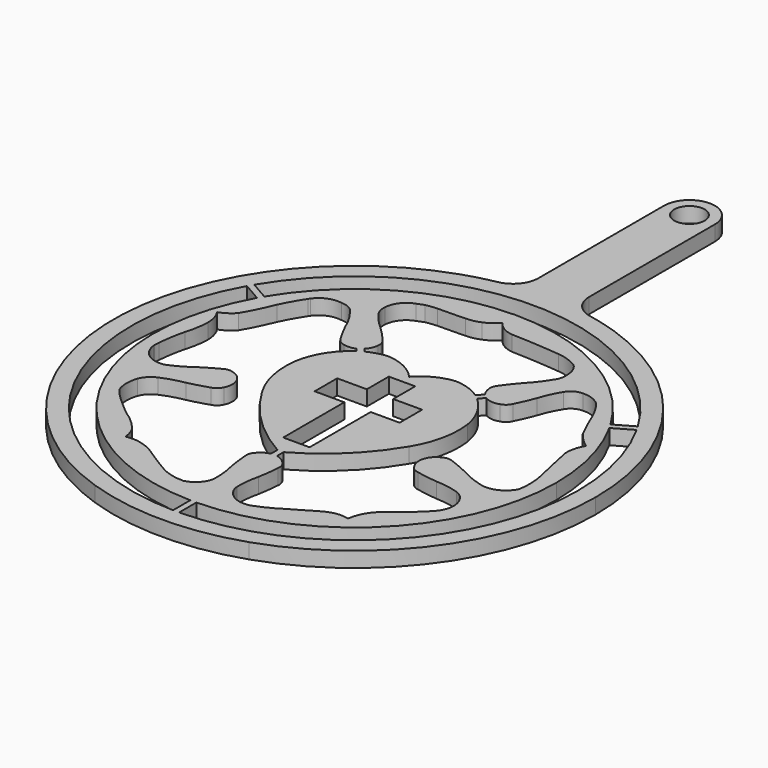
from build123d import *

# Parameters (mm, degrees)
F1_DEPTH = 3
F2_R     = 4.99999
F3_R     = 3
F4_DEPTH = 3.001


# Not quite as in the source:
# - a fillet or chamfer is up to 0.001 mm smaller than in the source, because OpenCascade refuses the exact size
# - a feature names something its author has since deleted; it is built from what else it names


with BuildPart() as f1:
    # F0 (on Top) → F1 (new body)
    with BuildSketch(Plane.XY):
        with BuildLine():
            Line((15.2069063257, 45), (-15.2069063257, 45))
            ThreePointArc((-15.2069063257, 45), (-33.5875721064, 33.5875721064), (-45, 15.2069063257))
            Line((-45, 15.2069063257), (-45, -15.2069063257))
            ThreePointArc((-45, -15.2069063257), (-33.5875721064, -33.5875721064), (-15.2069063257, -45))
            Line((-15.2069063257, -45), (15.2069063257, -45))
            ThreePointArc((15.2069063257, -45), (33.5875721064, -33.5875721064), (45, -15.2069063257))
            Line((45, -15.2069063257), (45, 15.2069063257))
            ThreePointArc((45, 15.2069063257), (33.5875721064, 33.5875721064), (15.2069063257, 45))
        make_face()
        with BuildLine():
            ThreePointArc((38.4015747706, 21.4783392081), (42.5773959391, 11.0979887839), (44, 0))
            ThreePointArc((44, 0), (31.3241121183, -30.8998381873), (0.6, -43.9959089007))
            ThreePointArc((0.6, -43.9959089007), (0, -44), (-0.6, -43.9959089007))
            ThreePointArc((-0.6, -43.9959089007), (-38.1051177665, -22), (-38.4015747706, 21.4783392081))
            ThreePointArc((-38.4015747706, 21.4783392081), (-38.1051177665, 22), (-37.8015747706, 22.5175696926))
            ThreePointArc((-37.8015747706, 22.5175696926), (0, 44), (37.8015747706, 22.5175696926))
            ThreePointArc((37.8015747706, 22.5175696926), (38.1051177665, 22), (38.4015747706, 21.4783392081))
        make_face(mode=Mode.SUBTRACT)
        with BuildLine():
            ThreePointArc((39.75, 0), (38.4721059413, 9.9979780177), (34.7205879526, 19.3531204778))
            ThreePointArc((34.7205879526, 19.3531204778), (34.4245098004, 19.875), (34.1205879526, 20.3923509623))
            ThreePointArc((34.1205879526, 20.3923509623), (0, 39.75), (-34.1205879526, 20.3923509623))
            ThreePointArc((-34.1205879526, 20.3923509623), (-34.4245098004, 19.875), (-34.7205879526, 19.3531204778))
            ThreePointArc((-34.7205879526, 19.3531204778), (-34.4245098004, -19.875), (-0.6, -39.7454714402))
            ThreePointArc((-0.6, -39.7454714402), (0, -39.75), (0.6, -39.7454714402))
            ThreePointArc((0.6, -39.7454714402), (28.3188320734, -27.8945559205), (39.75, 0))
        make_face()
        with BuildLine():
            ThreePointArc((13.1544303149, 18.6974834651), (12.9994836516, 17.710085626), (13.2698951604, 16.7478795269))
            ThreePointArc((13.2698951604, 16.7478795269), (13.6237788684, 16.2513300709), (14.0937424239, 15.8628338707))
            ThreePointArc((14.0937424239, 15.8628338707), (15.8973722034, 15.5715459018), (17.3623822629, 16.6631843895))
            ThreePointArc((17.3623822629, 16.6631843895), (18.3033011466, 18.6424294995), (19.0587975085, 20.6996034831))
            ThreePointArc((19.0587975085, 20.6996034831), (19.6962425586, 22.4376385334), (20.4611290246, 24.1234768182))
            ThreePointArc((20.4611290246, 24.1234768182), (21.7193319348, 25.6187652762), (23.5025491565, 26.4182016253))
            ThreePointArc((23.5025491565, 26.4182016253), (25.4580904224, 26.3810636918), (27.1545499563, 25.4076439887))
            ThreePointArc((27.1545499563, 25.4076439887), (27.52673708, 25.0168961336), (27.8844064433, 24.6128172206))
            ThreePointArc((27.8844064433, 24.6128172206), (29.2916671808, 22.6613798031), (30.363548547, 20.5074157566))
            ThreePointArc((30.363548547, 20.5074157566), (31.5171358074, 17.8349379562), (32.7894538641, 15.2169028297))
            ThreePointArc((32.7894538641, 15.2169028297), (34.1230277014, 13.7207168946), (35.6659889221, 12.4415522441))
            ThreePointArc((35.6659889221, 12.4415522441), (34.8647886426, 10.5924571906), (34.6556343138, 8.5881296545))
            ThreePointArc((34.6556343138, 8.5881296545), (35.5419764472, 4.3940722193), (36.4768467844, 0.2105644089))
            ThreePointArc((36.4768467844, 0.2105644089), (36.8063640413, -2.5236804449), (36.5942801272, -5.269531307))
            ThreePointArc((36.5942801272, -5.269531307), (36.5776420507, -5.3615212162), (36.5603901446, -5.4533979855))
            ThreePointArc((36.5603901446, -5.4533979855), (35.5463694507, -7.1539827552), (34.0106971562, -8.4037575871))
            ThreePointArc((34.0106971562, -8.4037575871), (32.5922946208, -8.674299863), (31.1614554375, -8.4799854085))
            ThreePointArc((31.1614554375, -8.4799854085), (27.7166740101, -7.1552393182), (24.3694968522, -5.6002871133))
            ThreePointArc((24.3694968522, -5.6002871133), (22.9198378539, -5.167220158), (21.4094873518, -5.2560996264))
            ThreePointArc((21.4094873518, -5.2560996264), (20.4460224679, -5.7761838724), (19.8262277991, -6.6787395626))
            ThreePointArc((19.8262277991, -6.6787395626), (19.6988373955, -7.9117885325), (20.3195624053, -8.9847929776))
            ThreePointArc((20.3195624053, -8.9847929776), (21.6411737408, -9.7871390742), (23.1533683836, -10.1091377437))
            ThreePointArc((23.1533683836, -10.1091377437), (25.0267759883, -10.2520123025), (26.8935356289, -10.4647977278))
            ThreePointArc((26.8935356289, -10.4647977278), (28.7622135844, -10.6241884707), (30.5648632348, -11.1416988075))
            ThreePointArc((30.5648632348, -11.1416988075), (31.9095412868, -12.2463559177), (32.7662372269, -13.7611161168))
            ThreePointArc((32.7662372269, -13.7611161168), (32.8659343413, -15.4387331126), (32.3565080762, -17.040239647))
            ThreePointArc((32.3565080762, -17.040239647), (31.9517024959, -17.7441363632), (31.4918024275, -18.4133374331))
            ThreePointArc((31.4918024275, -18.4133374331), (30.8813307917, -19.1535972301), (30.2035380155, -19.8327563703))
            ThreePointArc((30.2035380155, -19.8327563703), (28.6944924477, -21.2622272709), (27.0892698318, -22.5827824324))
            ThreePointArc((27.0892698318, -22.5827824324), (25.8109799054, -23.5447087894), (24.6124230325, -24.6043261141))
            ThreePointArc((24.6124230325, -24.6043261141), (23.0161745176, -26.6759411416), (22.1902150661, -29.1573498398))
            ThreePointArc((22.1902150661, -29.1573498398), (22.1823714034, -29.2604491115), (22.1902150661, -29.3635483831))
            ThreePointArc((22.1902150661, -29.3635483831), (20.6543600705, -29.1355721936), (19.1159117967, -29.3453354388))
            ThreePointArc((19.1159117967, -29.3453354388), (18.0140299323, -29.7476012069), (16.9789958745, -30.2995666862))
            ThreePointArc((16.9789958745, -30.2995666862), (14.8518935693, -31.5584511018), (12.7147845924, -32.8002721071))
            ThreePointArc((12.7147845924, -32.8002721071), (10.3373434694, -34.1802416761), (7.8145563602, -35.2720692754))
            ThreePointArc((7.8145563602, -35.2720692754), (4.7183466369, -35.6236947606), (1.902480959, -34.2891328037))
            ThreePointArc((1.902480959, -34.2891328037), (1.1117117622, -32.5153233248), (1.0741840815, -30.5735953152))
            ThreePointArc((1.0741840815, -30.5735953152), (1.4077427625, -27.3798938968), (1.8937365385, -24.2058113217))
            ThreePointArc((1.8937365385, -24.2058113217), (1.9589663636, -22.7965979751), (1.7485594144, -21.4016549289))
            ThreePointArc((1.7485594144, -21.4016549289), (1.3000904024, -20.7086359573), (0.6, -20.2712880658))
            ThreePointArc((0.6, -20.2712880658), (0.3043633322, -20.1930320032), (0, -20.1632324606))
            ThreePointArc((0, -20.1632324606), (-0.3001138701, -20.1435719399), (-0.6, -20.1664450732))
            ThreePointArc((-0.6, -20.1664450732), (-1.5074907875, -20.5274222481), (-2.1579356398, -21.2559588253))
            ThreePointArc((-2.1579356398, -21.2559588253), (-2.5611237062, -22.7415693157), (-2.4770193268, -24.278620258))
            ThreePointArc((-2.4770193268, -24.278620258), (-1.9152687902, -27.3259041519), (-1.5005924506, -30.3966607898))
            ThreePointArc((-1.5005924506, -30.3966607898), (-1.7771048177, -32.3321939483), (-2.8084376827, -33.9932478964))
            ThreePointArc((-2.8084376827, -33.9932478964), (-3.8656823021, -34.9221705279), (-5.2103865892, -35.3374220431))
            ThreePointArc((-5.2103865892, -35.3374220431), (-5.344161676, -35.3425806413), (-5.4779952594, -35.3458907678))
            ThreePointArc((-5.4779952594, -35.3458907678), (-7.7809432718, -35.1103947403), (-9.962332435, -34.3354307115))
            ThreePointArc((-9.962332435, -34.3354307115), (-12.6447845502, -32.7277147455), (-15.2711598203, -31.0299359262))
            ThreePointArc((-15.2711598203, -31.0299359262), (-16.8965931087, -30.0854125724), (-18.6754819006, -29.4773727655))
            ThreePointArc((-18.6754819006, -29.4773727655), (-20.163660707, -29.2771457572), (-21.6584373266, -29.4200088829))
            ThreePointArc((-21.6584373266, -29.4200088829), (-21.9469277164, -27.9249853374), (-22.6042401046, -26.551572606))
            ThreePointArc((-22.6042401046, -26.551572606), (-24.4508663247, -24.6630203424), (-26.5681687742, -23.0838786811))
            ThreePointArc((-26.5681687742, -23.0838786811), (-28.2946605833, -21.6202528417), (-29.9907564706, -20.1215089324))
            ThreePointArc((-29.9907564706, -20.1215089324), (-31.1955319716, -18.9227074216), (-32.2594381869, -17.5972970567))
            ThreePointArc((-32.2594381869, -17.5972970567), (-32.7127552743, -16.9261962228), (-33.1298090107, -16.2319780353))
            ThreePointArc((-33.1298090107, -16.2319780353), (-33.5060127096, -14.1649201538), (-33.1298090107, -12.0978622723))
            ThreePointArc((-33.1298090107, -12.0978622723), (-31.9416458989, -10.6809065614), (-30.2762478179, -9.8771999615))
            ThreePointArc((-30.2762478179, -9.8771999615), (-27.3934880183, -9.0605324957), (-24.4824323392, -8.3513042915))
            ThreePointArc((-24.4824323392, -8.3513042915), (-22.8843269804, -7.9189260706), (-21.4011013097, -7.1834444094))
            ThreePointArc((-21.4011013097, -7.1834444094), (-20.6895055917, -6.0012895415), (-20.7867655492, -4.6249178263))
            ThreePointArc((-20.7867655492, -4.6249178263), (-21.7066659737, -3.4710484078), (-23.1462172753, -3.1465126227))
            ThreePointArc((-23.1462172753, -3.1465126227), (-25.0854890454, -3.7516390034), (-26.8341671265, -4.7856012385))
            ThreePointArc((-26.8341671265, -4.7856012385), (-28.4361773324, -5.8823391866), (-30.0850268043, -6.9073105256))
            ThreePointArc((-30.0850268043, -6.9073105256), (-31.4989957357, -7.5753525343), (-33.0535970218, -7.7450673121))
            ThreePointArc((-33.0535970218, -7.7450673121), (-34.8285220711, -7.3095151895), (-36.249821592, -6.1606147352))
            ThreePointArc((-36.249821592, -6.1606147352), (-36.9862452296, -4.5062677921), (-37.2370698922, -2.7128714134))
            ThreePointArc((-37.2370698922, -2.7128714134), (-37.2194603589, -2.241264003), (-37.167636264, -1.7721820182))
            ThreePointArc((-37.167636264, -1.7721820182), (-36.8335814434, 0.9244367586), (-36.2805403358, 3.584792183))
            ThreePointArc((-36.2805403358, 3.584792183), (-35.7282804227, 5.8900650394), (-35.5035714394, 8.2498912674))
            ThreePointArc((-35.5035714394, 8.2498912674), (-35.7673793213, 10.0960235572), (-36.5443281419, 11.7913552535))
            ThreePointArc((-36.5443281419, 11.7913552535), (-35.0440824364, 12.526502069), (-33.7808481938, 13.6198534605))
            ThreePointArc((-33.7808481938, 13.6198534605), (-32.2465790302, 16.4891609765), (-30.9187691248, 19.4596539226))
            ThreePointArc((-30.9187691248, 19.4596539226), (-29.7224672012, 21.7811291171), (-28.3643565353, 24.0118063215))
            ThreePointArc((-28.3643565353, 24.0118063215), (-28.2608924895, 24.1742639387), (-28.1508342247, 24.3323286865))
            ThreePointArc((-28.1508342247, 24.3323286865), (-27.9161509949, 24.6764245366), (-27.6775840259, 25.017839202))
            ThreePointArc((-27.6775840259, 25.017839202), (-26.0121072138, 26.4235192892), (-23.9492948688, 27.1267651555))
            ThreePointArc((-23.9492948688, 27.1267651555), (-22.683343624, 27.1559317042), (-21.4851997382, 26.7461336193))
            ThreePointArc((-21.4851997382, 26.7461336193), (-20.2944890997, 25.6536896702), (-19.3477306104, 24.3441577044))
            ThreePointArc((-19.3477306104, 24.3441577044), (-18.1261905857, 22.1694079096), (-16.9467623866, 19.9715348867))
            ThreePointArc((-16.9467623866, 19.9715348867), (-16.124822625, 18.3782931612), (-14.9433059207, 17.0299525347))
            ThreePointArc((-14.9433059207, 17.0299525347), (-13.9414482308, 16.5529147578), (-12.8357349956, 16.6460926139))
            ThreePointArc((-12.8357349956, 16.6460926139), (-12.432827299, 16.8427191161), (-12.0801559116, 17.1195213667))
            ThreePointArc((-12.0801559116, 17.1195213667), (-11.9641864634, 17.2253159453), (-11.855745386, 17.338814573))
            ThreePointArc((-11.855745386, 17.338814573), (-11.3489235944, 18.28613132), (-11.3304612786, 19.3603456797))
            ThreePointArc((-11.3304612786, 19.3603456797), (-11.6131657763, 20.0806167396), (-12.0245722681, 20.7359463753))
            ThreePointArc((-12.0245722681, 20.7359463753), (-13.0298005438, 21.9109290811), (-14.1447644308, 22.9823411287))
            ThreePointArc((-14.1447644308, 22.9823411287), (-15.2704276162, 23.960127427), (-16.3859091699, 24.9495133758))
            ThreePointArc((-16.3859091699, 24.9495133758), (-17.420474299, 26.17199909), (-18.1667581201, 27.588987723))
            ThreePointArc((-18.1667581201, 27.588987723), (-18.4111606757, 29.1457914028), (-18.0553290993, 30.6809637696))
            ThreePointArc((-18.0553290993, 30.6809637696), (-17.0147657832, 32.084699542), (-15.5111001804, 32.9747758806))
            ThreePointArc((-15.5111001804, 32.9747758806), (-14.3049296056, 33.3550786383), (-13.0737277589, 33.6442492729))
            ThreePointArc((-13.0737277589, 33.6442492729), (-11.9572647742, 33.8243078309), (-10.8312694356, 33.9294038713))
            ThreePointArc((-10.8312694356, 33.9294038713), (-8.1108956333, 33.9565345059), (-5.3912550211, 34.0252704918))
            ThreePointArc((-5.3912550211, 34.0252704918), (-3.9483394584, 34.1858040453), (-2.5609757286, 34.6135869622))
            ThreePointArc((-2.5609757286, 34.6135869622), (-1.1721033451, 35.3723533238), (0, 36.4357754588))
            ThreePointArc((0, 36.4357754588), (1.5528861369, 34.9900948734), (3.5677228589, 34.3253538013))
            ThreePointArc((3.5677228589, 34.3253538013), (8.4012669361, 34.1107132353), (13.2236303762, 33.7182469666))
            ThreePointArc((13.2236303762, 33.7182469666), (15.3400282605, 33.2604879218), (17.2954601791, 32.3304506325))
            ThreePointArc((17.2954601791, 32.3304506325), (17.6949809728, 32.0658775644), (18.0804952979, 31.7812822759))
            ThreePointArc((18.0804952979, 31.7812822759), (19.0718846436, 30.3757755061), (19.5259880275, 28.7168323994))
            ThreePointArc((19.5259880275, 28.7168323994), (18.9871091632, 26.7721210867), (17.8583189845, 25.0993613154))
            Line((17.8583189845, 25.0993613154), (15.5178485438, 22.0934618264))
            ThreePointArc((15.5178485438, 22.0934618264), (14.1512044305, 20.5241774551), (13.1544303149, 18.6974834651))
        make_face(mode=Mode.SUBTRACT)
        with BuildLine():
            Line((-5, 87.5), (-5, 47.2361090692))
            ThreePointArc((-5, 47.2361090692), (0, 47.5), (5, 47.2361090692))
            Line((5, 47.2361090692), (5, 87.5))
            Line((5, 87.5), (-5, 87.5))
        make_face()
        with BuildLine():
            Line((-2.4924513418, 6.1171003617), (-2.4924513418, 11.5402890369))
            Line((-2.4924513418, 11.5402890369), (0, 11.5402890369))
            Line((0, 11.5402890369), (0, 13.4395202622))
            ThreePointArc((0, 13.4395202622), (-2.9522200359, 15.7305615155), (-6.5359184518, 16.7896077037))
            ThreePointArc((-6.5359184518, 16.7896077037), (-8.6542895394, 16.4571090738), (-10.6554259019, 15.6867165363))
            ThreePointArc((-10.6554259019, 15.6867165363), (-11.1837139042, 15.3959685754), (-11.6937909943, 15.0743415363))
            ThreePointArc((-11.6937909943, 15.0743415363), (-11.8463732448, 14.9696339693), (-11.9970198721, 14.8621601984))
            ThreePointArc((-11.9970198721, 14.8621601984), (-15.269507602, 11.1829402277), (-16.9533155859, 6.5557784401))
            ThreePointArc((-16.9533155859, 6.5557784401), (-16.6901469812, 0.6933904938), (-14.4818136469, -4.7435308807))
            ThreePointArc((-14.4818136469, -4.7435308807), (-8.4346309374, -12.4175447977), (-0.6, -18.2551356018))
            ThreePointArc((-0.6, -18.2551356018), (-0.3007512971, -18.4202689289), (0, -18.582649529))
            Line((0, -18.582649529), (0, -14.4816143438))
            Line((0, -14.4816143438), (-2.4924513418, -14.4816143438))
            Line((-2.4924513418, -14.4816143438), (-2.4924513418, 0.5696658045))
            Line((-2.4924513418, 0.5696658045), (-8.3385352045, 0.5696658045))
            Line((-8.3385352045, 0.5696658045), (-8.3385352045, 6.1171003617))
            Line((-8.3385352045, 6.1171003617), (-2.4924513418, 6.1171003617))
        make_face()
        with BuildLine():
            Line((0, 13.4395202622), (0, 11.5402890369))
            Line((0, 11.5402890369), (2.7075468097, 11.5402890369))
            Line((2.7075468097, 11.5402890369), (2.7075468097, 6.1171003617))
            Line((2.7075468097, 6.1171003617), (8.4134116769, 6.1171003617))
            Line((8.4134116769, 6.1171003617), (8.4134116769, 0.5696658045))
            Line((8.4134116769, 0.5696658045), (2.7075468097, 0.5696658045))
            Line((2.7075468097, 0.5696658045), (2.7075468097, -14.4816143438))
            Line((2.7075468097, -14.4816143438), (0, -14.4816143438))
            Line((0, -14.4816143438), (0, -18.582649529))
            ThreePointArc((0, -18.582649529), (0.3007512971, -18.4202689289), (0.6, -18.2551356018))
            ThreePointArc((0.6, -18.2551356018), (8.4346309374, -12.4175447977), (14.4818136469, -4.7435308807))
            ThreePointArc((14.4818136469, -4.7435308807), (16.6901469812, 0.6933904938), (16.9533155859, 6.5557784401))
            ThreePointArc((16.9533155859, 6.5557784401), (15.5086264172, 10.7649279062), (12.7387291979, 14.2479919906))
            ThreePointArc((12.7387291979, 14.2479919906), (12.3735173621, 14.5618907382), (11.9970198721, 14.8621601984))
            ThreePointArc((11.9970198721, 14.8621601984), (11.9004435295, 14.9315356124), (11.8030605273, 14.9997740831))
            ThreePointArc((11.8030605273, 14.9997740831), (9.2945898699, 16.2628376694), (6.5359184518, 16.7896077037))
            ThreePointArc((6.5359184518, 16.7896077037), (2.9522200359, 15.7305615155), (0, 13.4395202622))
        make_face()
        with BuildLine():
            Line((-45, -15.2069063257), (-45, 15.2069063257))
            ThreePointArc((-45, 15.2069063257), (-47.5, 0), (-45, -15.2069063257))
        make_face()
        with BuildLine():
            ThreePointArc((47.5, 0), (46.8708331481, 7.7055175037), (45, 15.2069063257))
            Line((45, 15.2069063257), (45, -15.2069063257))
            ThreePointArc((45, -15.2069063257), (46.8708331481, -7.7055175037), (47.5, 0))
        make_face()
        with BuildLine():
            ThreePointArc((-5, 47.2361090692), (-10.1651272376, 46.399570992), (-15.2069063257, 45))
            Line((-15.2069063257, 45), (15.2069063257, 45))
            ThreePointArc((15.2069063257, 45), (10.1651272376, 46.399570992), (5, 47.2361090692))
            ThreePointArc((5, 47.2361090692), (0, 47.5), (-5, 47.2361090692))
        make_face()
        with BuildLine():
            Line((15.2069063257, -45), (-15.2069063257, -45))
            ThreePointArc((-15.2069063257, -45), (0, -47.5), (15.2069063257, -45))
        make_face()
        with BuildLine():
            Line((-37.2028201905, -3.0520430721), (-37.2370698922, -2.7128714134))
            ThreePointArc((-37.2370698922, -2.7128714134), (-36.9862452296, -4.5062677921), (-36.249821592, -6.1606147352))
            ThreePointArc((-36.249821592, -6.1606147352), (-34.8285220711, -7.3095151895), (-33.0535970218, -7.7450673121))
            ThreePointArc((-33.0535970218, -7.7450673121), (-31.4989957357, -7.5753525343), (-30.0850268043, -6.9073105256))
            ThreePointArc((-30.0850268043, -6.9073105256), (-28.4361773324, -5.8823391866), (-26.8341671265, -4.7856012385))
            ThreePointArc((-26.8341671265, -4.7856012385), (-25.0854890454, -3.7516390034), (-23.1462172753, -3.1465126227))
            ThreePointArc((-23.1462172753, -3.1465126227), (-21.7066659737, -3.4710484078), (-20.7867655492, -4.6249178263))
            ThreePointArc((-20.7867655492, -4.6249178263), (-20.6895055917, -6.0012895415), (-21.4011013097, -7.1834444094))
            ThreePointArc((-21.4011013097, -7.1834444094), (-22.8843269804, -7.9189260706), (-24.4824323392, -8.3513042915))
            ThreePointArc((-24.4824323392, -8.3513042915), (-27.3934880183, -9.0605324957), (-30.2762478179, -9.8771999615))
            ThreePointArc((-30.2762478179, -9.8771999615), (-31.9416458989, -10.6809065614), (-33.1298090107, -12.0978622723))
            ThreePointArc((-33.1298090107, -12.0978622723), (-33.5060127096, -14.1649201538), (-33.1298090107, -16.2319780353))
            ThreePointArc((-33.1298090107, -16.2319780353), (-32.7127552743, -16.9261962228), (-32.2594381869, -17.5972970567))
            ThreePointArc((-32.2594381869, -17.5972970567), (-32.6321128417, -15.3758618232), (-32.2594381869, -13.1544265896))
            ThreePointArc((-32.2594381869, -13.1544265896), (-31.3761557144, -11.7768380517), (-30.011004529, -10.8744521324))
            ThreePointArc((-30.011004529, -10.8744521324), (-27.829629741, -10.0706684601), (-25.5653052745, -9.5440767125))
            ThreePointArc((-25.5653052745, -9.5440767125), (-23.545938443, -9.0389737836), (-21.558195876, -8.421032964))
            ThreePointArc((-21.558195876, -8.421032964), (-20.6612270025, -7.9549542831), (-20.0762329553, -7.1305972844))
            ThreePointArc((-20.0762329553, -7.1305972844), (-19.9343099504, -4.2114197585), (-22.1327785323, -2.2856795213))
            ThreePointArc((-22.1327785323, -2.2856795213), (-23.1321423428, -2.133842533), (-24.0904982241, -2.4553024864))
            ThreePointArc((-24.0904982241, -2.4553024864), (-25.9158096623, -3.4559070648), (-27.6819203749, -4.5576440207))
            ThreePointArc((-27.6819203749, -4.5576440207), (-29.6336507215, -5.8206613651), (-31.7271545635, -6.8314560136))
            ThreePointArc((-31.7271545635, -6.8314560136), (-32.880737006, -7.0189670856), (-34.0351934379, -6.8369143444))
            ThreePointArc((-34.0351934379, -6.8369143444), (-36.2004795426, -5.4311236792), (-37.2028201905, -3.0520430721))
        make_face()
        with BuildLine():
            ThreePointArc((36.5603901446, -5.4533979855), (36.5776420507, -5.3615212162), (36.5942801272, -5.269531307))
            ThreePointArc((36.5942801272, -5.269531307), (35.4829664149, -6.702693278), (33.923342824, -7.6281907968))
            ThreePointArc((33.923342824, -7.6281907968), (32.3863989761, -7.9398839226), (30.8351305224, -7.7098509235))
            ThreePointArc((30.8351305224, -7.7098509235), (28.6315485295, -6.9691144259), (26.5370464456, -5.9603898955))
            ThreePointArc((26.5370464456, -5.9603898955), (24.6468956359, -5.0884373246), (22.7106715987, -4.3242332637))
            ThreePointArc((22.7106715987, -4.3242332637), (21.7196099075, -4.1252879925), (20.7471193152, -4.4010497461))
            ThreePointArc((20.7471193152, -4.4010497461), (18.807050081, -6.5868838966), (19.313334855, -9.4653236292))
            ThreePointArc((19.313334855, -9.4653236292), (19.9969347297, -10.2099535427), (20.9451985667, -10.5600652281))
            ThreePointArc((20.9451985667, -10.5600652281), (22.9946664974, -10.9242802335), (25.0613826562, -11.1725858678))
            ThreePointArc((25.0613826562, -11.1725858678), (27.3738194149, -11.4115427573), (29.63866336, -11.9358957513))
            ThreePointArc((29.63866336, -11.9358957513), (30.655111141, -12.5127378113), (31.4406309573, -13.3781114138))
            ThreePointArc((31.4406309573, -13.3781114138), (32.2469153329, -15.8305829866), (31.5370009593, -18.3126653567))
            Line((31.5370009593, -18.3126653567), (31.4918024275, -18.4133374331))
            ThreePointArc((31.4918024275, -18.4133374331), (31.9517024959, -17.7441363632), (32.3565080762, -17.040239647))
            ThreePointArc((32.3565080762, -17.040239647), (32.8659343413, -15.4387331126), (32.7662372269, -13.7611161168))
            ThreePointArc((32.7662372269, -13.7611161168), (31.9095412868, -12.2463559177), (30.5648632348, -11.1416988075))
            ThreePointArc((30.5648632348, -11.1416988075), (28.7622135844, -10.6241884707), (26.8935356289, -10.4647977278))
            ThreePointArc((26.8935356289, -10.4647977278), (25.0267759883, -10.2520123025), (23.1533683836, -10.1091377437))
            ThreePointArc((23.1533683836, -10.1091377437), (21.6411737408, -9.7871390742), (20.3195624053, -8.9847929776))
            ThreePointArc((20.3195624053, -8.9847929776), (19.6988373955, -7.9117885325), (19.8262277991, -6.6787395626))
            ThreePointArc((19.8262277991, -6.6787395626), (20.4460224679, -5.7761838724), (21.4094873518, -5.2560996264))
            ThreePointArc((21.4094873518, -5.2560996264), (22.9198378539, -5.167220158), (24.3694968522, -5.6002871133))
            ThreePointArc((24.3694968522, -5.6002871133), (27.7166740101, -7.1552393182), (31.1614554375, -8.4799854085))
            ThreePointArc((31.1614554375, -8.4799854085), (32.5922946208, -8.674299863), (34.0106971562, -8.4037575871))
            ThreePointArc((34.0106971562, -8.4037575871), (35.5463694507, -7.1539827552), (36.5603901446, -5.4533979855))
        make_face()
        with BuildLine():
            ThreePointArc((2.6316633448, -21.1005806923), (1.726653252, -20.3069906412), (0.6, -19.8833387949))
            Line((0.6, -19.8833387949), (0.6, -20.2712880658))
            ThreePointArc((0.6, -20.2712880658), (1.3000904024, -20.7086359573), (1.7485594144, -21.4016549289))
            ThreePointArc((1.7485594144, -21.4016549289), (1.9589663636, -22.7965979751), (1.8937365385, -24.2058113217))
            ThreePointArc((1.8937365385, -24.2058113217), (1.4077427625, -27.3798938968), (1.0741840815, -30.5735953152))
            ThreePointArc((1.0741840815, -30.5735953152), (1.1117117622, -32.5153233248), (1.902480959, -34.2891328037))
            ThreePointArc((1.902480959, -34.2891328037), (4.7183466369, -35.6236947606), (7.8145563602, -35.2720692754))
            ThreePointArc((7.8145563602, -35.2720692754), (5.2329554221, -35.2789906946), (3.0928736087, -33.8351204991))
            ThreePointArc((3.0928736087, -33.8351204991), (2.4742111124, -32.8435714235), (2.1960753947, -31.7084267735))
            ThreePointArc((2.1960753947, -31.7084267735), (2.3085196558, -29.3863973926), (2.7085314505, -27.0963199437))
            ThreePointArc((2.7085314505, -27.0963199437), (3.0326112339, -25.0401235369), (3.2404666066, -22.9689481428))
            ThreePointArc((3.2404666066, -22.9689481428), (3.1619125789, -21.9611724924), (2.6316633448, -21.1005806923))
        make_face()
        with BuildLine():
            ThreePointArc((-14.5316705152, 15.5238754682), (-13.3330414416, 15.413799216), (-12.1725435066, 15.7332878386))
            Line((-12.1725435066, 15.7332878386), (-12.8357349956, 16.6460926139))
            ThreePointArc((-12.8357349956, 16.6460926139), (-13.9414482308, 16.5529147578), (-14.9433059207, 17.0299525347))
            ThreePointArc((-14.9433059207, 17.0299525347), (-16.124822625, 18.3782931612), (-16.9467623866, 19.9715348867))
            ThreePointArc((-16.9467623866, 19.9715348867), (-18.1261905857, 22.1694079096), (-19.3477306104, 24.3441577044))
            ThreePointArc((-19.3477306104, 24.3441577044), (-20.2944890997, 25.6536896702), (-21.4851997382, 26.7461336193))
            ThreePointArc((-21.4851997382, 26.7461336193), (-22.683343624, 27.1559317042), (-23.9492948688, 27.1267651555))
            ThreePointArc((-23.9492948688, 27.1267651555), (-26.0121072138, 26.4235192892), (-27.6775840259, 25.017839202))
            ThreePointArc((-27.6775840259, 25.017839202), (-27.9161509949, 24.6764245366), (-28.1508342247, 24.3323286865))
            ThreePointArc((-28.1508342247, 24.3323286865), (-26.1026850154, 25.925821232), (-23.5205199569, 26.1838082224))
            ThreePointArc((-23.5205199569, 26.1838082224), (-21.7195681497, 25.6954363041), (-20.4144079462, 24.3618353947))
            ThreePointArc((-20.4144079462, 24.3618353947), (-19.1405226388, 22.4171810857), (-18.1180652275, 20.3293484775))
            ThreePointArc((-18.1180652275, 20.3293484775), (-17.1716493561, 18.4753613234), (-16.1224015335, 16.6775709085))
            ThreePointArc((-16.1224015335, 16.6775709085), (-15.4664943252, 15.9084361799), (-14.5316705152, 15.5238754682))
        make_face()
        with BuildLine():
            Line((-11.855745386, 17.338814573), (-11.2017231134, 16.4386301414))
            ThreePointArc((-11.2017231134, 16.4386301414), (-10.5392577931, 17.4436018507), (-10.2735497763, 18.6175812743))
            ThreePointArc((-10.2735497763, 18.6175812743), (-10.3504123031, 19.6254873457), (-10.8792164246, 20.4869678723))
            ThreePointArc((-10.8792164246, 20.4869678723), (-12.264781305, 22.0404096418), (-13.735569281, 23.5134181614))
            ThreePointArc((-13.735569281, 23.5134181614), (-15.405259372, 25.1310087024), (-16.8610833156, 26.9434768547))
            ThreePointArc((-16.8610833156, 26.9434768547), (-17.3032880778, 28.0253122405), (-17.385597528, 29.1911329849))
            ThreePointArc((-17.385597528, 29.1911329849), (-16.5029205787, 31.6171570394), (-14.410293239, 33.1289844523))
            Line((-14.410293239, 33.1289844523), (-13.0737277589, 33.6442492729))
            ThreePointArc((-13.0737277589, 33.6442492729), (-14.3049296056, 33.3550786383), (-15.5111001804, 32.9747758806))
            ThreePointArc((-15.5111001804, 32.9747758806), (-17.0147657832, 32.084699542), (-18.0553290993, 30.6809637696))
            ThreePointArc((-18.0553290993, 30.6809637696), (-18.4111606757, 29.1457914028), (-18.1667581201, 27.588987723))
            ThreePointArc((-18.1667581201, 27.588987723), (-17.420474299, 26.17199909), (-16.3859091699, 24.9495133758))
            ThreePointArc((-16.3859091699, 24.9495133758), (-15.2704276162, 23.960127427), (-14.1447644308, 22.9823411287))
            ThreePointArc((-14.1447644308, 22.9823411287), (-13.0298005438, 21.9109290811), (-12.0245722681, 20.7359463753))
            ThreePointArc((-12.0245722681, 20.7359463753), (-11.6131657763, 20.0806167396), (-11.3304612786, 19.3603456797))
            ThreePointArc((-11.3304612786, 19.3603456797), (-11.3489235944, 18.28613132), (-11.855745386, 17.338814573))
        make_face()
        with BuildLine():
            Line((14.0937424239, 15.8628338707), (13.6631087202, 15.3496246071))
            ThreePointArc((13.6631087202, 15.3496246071), (15.1137877371, 14.8489258806), (16.6357861944, 15.0456223998))
            ThreePointArc((16.6357861944, 15.0456223998), (17.5335360432, 15.5101950054), (18.119912818, 16.3335690242))
            ThreePointArc((18.119912818, 16.3335690242), (19.008480177, 18.215966277), (19.7897090228, 20.1453840285))
            ThreePointArc((19.7897090228, 20.1453840285), (20.6263090732, 22.3143848384), (21.7258590717, 24.3626655708))
            ThreePointArc((21.7258590717, 24.3626655708), (22.851552613, 25.4542105558), (24.3737418205, 25.8305035532))
            ThreePointArc((24.3737418205, 25.8305035532), (26.2399373263, 25.5412857981), (27.8844064433, 24.6128172206))
            ThreePointArc((27.8844064433, 24.6128172206), (27.52673708, 25.0168961336), (27.1545499563, 25.4076439887))
            ThreePointArc((27.1545499563, 25.4076439887), (25.4580904224, 26.3810636918), (23.5025491565, 26.4182016253))
            ThreePointArc((23.5025491565, 26.4182016253), (21.7193319348, 25.6187652762), (20.4611290246, 24.1234768182))
            ThreePointArc((20.4611290246, 24.1234768182), (19.6962425586, 22.4376385334), (19.0587975085, 20.6996034831))
            ThreePointArc((19.0587975085, 20.6996034831), (18.3033011466, 18.6424294995), (17.3623822629, 16.6631843895))
            ThreePointArc((17.3623822629, 16.6631843895), (15.8973722034, 15.5715459018), (14.0937424239, 15.8628338707))
        make_face()
        with BuildLine():
            ThreePointArc((12.1242346632, 17.7564360457), (12.3471763961, 16.9164725799), (12.778113958, 16.1617975121))
            Line((12.778113958, 16.1617975121), (13.2698951604, 16.7478795269))
            ThreePointArc((13.2698951604, 16.7478795269), (12.9994836516, 17.710085626), (13.1544303149, 18.6974834651))
            ThreePointArc((13.1544303149, 18.6974834651), (14.1512044305, 20.5241774551), (15.5178485438, 22.0934618264))
            Line((15.5178485438, 22.0934618264), (17.8583189845, 25.0993613154))
            ThreePointArc((17.8583189845, 25.0993613154), (18.9871091632, 26.7721210867), (19.5259880275, 28.7168323994))
            ThreePointArc((19.5259880275, 28.7168323994), (19.0718846436, 30.3757755061), (18.0804952979, 31.7812822759))
            ThreePointArc((18.0804952979, 31.7812822759), (17.6949809728, 32.0658775644), (17.2954601791, 32.3304506325))
            ThreePointArc((17.2954601791, 32.3304506325), (18.269453025, 30.8662422437), (18.5829848051, 29.1358474642))
            ThreePointArc((18.5829848051, 29.1358474642), (18.527255018, 27.8171023277), (17.9610510352, 26.6247904582))
            ThreePointArc((17.9610510352, 26.6247904582), (16.6687339492, 24.6923358773), (15.1463798382, 22.9353776767))
            ThreePointArc((15.1463798382, 22.9353776767), (13.8095698061, 21.3397867807), (12.5646687896, 19.6714963899))
            ThreePointArc((12.5646687896, 19.6714963899), (12.1129599025, 18.7672057408), (12.1242346632, 17.7564360457))
        make_face()
        with BuildLine():
            Line((-0.6, -20.1664450732), (-0.6, -19.8833387949))
            ThreePointArc((-0.6, -19.8833387949), (-1.726653252, -20.3069906412), (-2.6316633448, -21.1005806923))
            ThreePointArc((-2.6316633448, -21.1005806923), (-3.1619125789, -21.9611724924), (-3.2404666066, -22.9689481428))
            ThreePointArc((-3.2404666066, -22.9689481428), (-3.0326112339, -25.0401235369), (-2.7085314505, -27.0963199437))
            ThreePointArc((-2.7085314505, -27.0963199437), (-2.3085196558, -29.3863973926), (-2.1960753947, -31.7084267735))
            ThreePointArc((-2.1960753947, -31.7084267735), (-2.4742111124, -32.8435714235), (-3.0928736087, -33.8351204991))
            ThreePointArc((-3.0928736087, -33.8351204991), (-4.1608134719, -34.7872504074), (-5.4779952594, -35.3458907678))
            ThreePointArc((-5.4779952594, -35.3458907678), (-5.344161676, -35.3425806413), (-5.2103865892, -35.3374220431))
            ThreePointArc((-5.2103865892, -35.3374220431), (-3.8656823021, -34.9221705279), (-2.8084376827, -33.9932478964))
            ThreePointArc((-2.8084376827, -33.9932478964), (-1.7771048177, -32.3321939483), (-1.5005924506, -30.3966607898))
            ThreePointArc((-1.5005924506, -30.3966607898), (-1.9152687902, -27.3259041519), (-2.4770193268, -24.278620258))
            ThreePointArc((-2.4770193268, -24.278620258), (-2.5611237062, -22.7415693157), (-2.1579356398, -21.2559588253))
            ThreePointArc((-2.1579356398, -21.2559588253), (-1.5074907875, -20.5274222481), (-0.6, -20.1664450732))
        make_face()
        with BuildLine():
            ThreePointArc((-0.6, -43.9959089007), (0, -44), (0.6, -43.9959089007))
            Line((0.6, -43.9959089007), (0.6, -39.7454714402))
            ThreePointArc((0.6, -39.7454714402), (0, -39.75), (-0.6, -39.7454714402))
            Line((-0.6, -39.7454714402), (-0.6, -43.9959089007))
        make_face()
        with BuildLine():
            Line((34.7205879526, 19.3531204778), (38.4015747706, 21.4783392081))
            ThreePointArc((38.4015747706, 21.4783392081), (38.1051177665, 22), (37.8015747706, 22.5175696926))
            Line((37.8015747706, 22.5175696926), (34.1205879526, 20.3923509623))
            ThreePointArc((34.1205879526, 20.3923509623), (34.4245098004, 19.875), (34.7205879526, 19.3531204778))
        make_face()
        with BuildLine():
            Line((-34.1205879526, 20.3923509623), (-37.8015747706, 22.5175696926))
            ThreePointArc((-37.8015747706, 22.5175696926), (-38.1051177665, 22), (-38.4015747706, 21.4783392081))
            Line((-38.4015747706, 21.4783392081), (-34.7205879526, 19.3531204778))
            ThreePointArc((-34.7205879526, 19.3531204778), (-34.4245098004, 19.875), (-34.1205879526, 20.3923509623))
        make_face()
        with BuildLine():
            Line((12.778113958, 16.1617975121), (11.8030605273, 14.9997740831))
            ThreePointArc((11.8030605273, 14.9997740831), (11.9004435295, 14.9315356124), (11.9970198721, 14.8621601984))
            ThreePointArc((11.9970198721, 14.8621601984), (12.3735173621, 14.5618907382), (12.7387291979, 14.2479919906))
            Line((12.7387291979, 14.2479919906), (13.6631087202, 15.3496246071))
            ThreePointArc((13.6631087202, 15.3496246071), (13.184018507, 15.7158372045), (12.778113958, 16.1617975121))
        make_face()
        with BuildLine():
            ThreePointArc((0.6, -18.2551356018), (0.3007512971, -18.4202689289), (0, -18.582649529))
            ThreePointArc((0, -18.582649529), (-0.3007512971, -18.4202689289), (-0.6, -18.2551356018))
            Line((-0.6, -18.2551356018), (-0.6, -19.8833387949))
            ThreePointArc((-0.6, -19.8833387949), (0, -19.8293263485), (0.6, -19.8833387949))
            Line((0.6, -19.8833387949), (0.6, -18.2551356018))
        make_face()
        with BuildLine():
            ThreePointArc((-12.1725435066, 15.7332878386), (-11.6553855905, 16.0422620029), (-11.2017231134, 16.4386301414))
            Line((-11.2017231134, 16.4386301414), (-11.855745386, 17.338814573))
            ThreePointArc((-11.855745386, 17.338814573), (-11.9641864634, 17.2253159453), (-12.0801559116, 17.1195213667))
            ThreePointArc((-12.0801559116, 17.1195213667), (-12.432827299, 16.8427191161), (-12.8357349956, 16.6460926139))
            Line((-12.8357349956, 16.6460926139), (-12.1725435066, 15.7332878386))
        make_face()
        with BuildLine():
            ThreePointArc((-11.6937909943, 15.0743415363), (-11.1837139042, 15.3959685754), (-10.6554259019, 15.6867165363))
            Line((-10.6554259019, 15.6867165363), (-11.2017231134, 16.4386301414))
            ThreePointArc((-11.2017231134, 16.4386301414), (-11.6553855905, 16.0422620029), (-12.1725435066, 15.7332878386))
            Line((-12.1725435066, 15.7332878386), (-11.6937909943, 15.0743415363))
        make_face()
        with BuildLine():
            Line((13.2698951604, 16.7478795269), (12.778113958, 16.1617975121))
            ThreePointArc((12.778113958, 16.1617975121), (13.184018507, 15.7158372045), (13.6631087202, 15.3496246071))
            Line((13.6631087202, 15.3496246071), (14.0937424239, 15.8628338707))
            ThreePointArc((14.0937424239, 15.8628338707), (13.6237788684, 16.2513300709), (13.2698951604, 16.7478795269))
        make_face()
        with BuildLine():
            Line((0.6, -20.2712880658), (0.6, -19.8833387949))
            ThreePointArc((0.6, -19.8833387949), (0, -19.8293263485), (-0.6, -19.8833387949))
            Line((-0.6, -19.8833387949), (-0.6, -20.1664450732))
            ThreePointArc((-0.6, -20.1664450732), (-0.3001138701, -20.1435719399), (0, -20.1632324606))
            ThreePointArc((0, -20.1632324606), (0.3043633322, -20.1930320032), (0.6, -20.2712880658))
        make_face()
    extrude(amount=F1_DEPTH)

    # F2 (radius 5 in the source; OpenCascade refuses exactly that, so slightly less here)
    f2_edges = [f1.edges().sort_by_distance(p)[0] for p in [
        (5, 47.236109, 1.5),
        (-5, 47.236109, 1.5),
        (-5, 87.5, 1.5),
        (5, 87.5, 1.5),
    ]]
    fillet(f2_edges, radius=F2_R)

    # F3 (on face) → F4 (cut, through all)
    with BuildSketch(Plane.XY.offset(3)):
        with Locations((0, 82.5)):
            Circle(F3_R)
    extrude(amount=-F4_DEPTH, mode=Mode.SUBTRACT)


solid = f1.part
